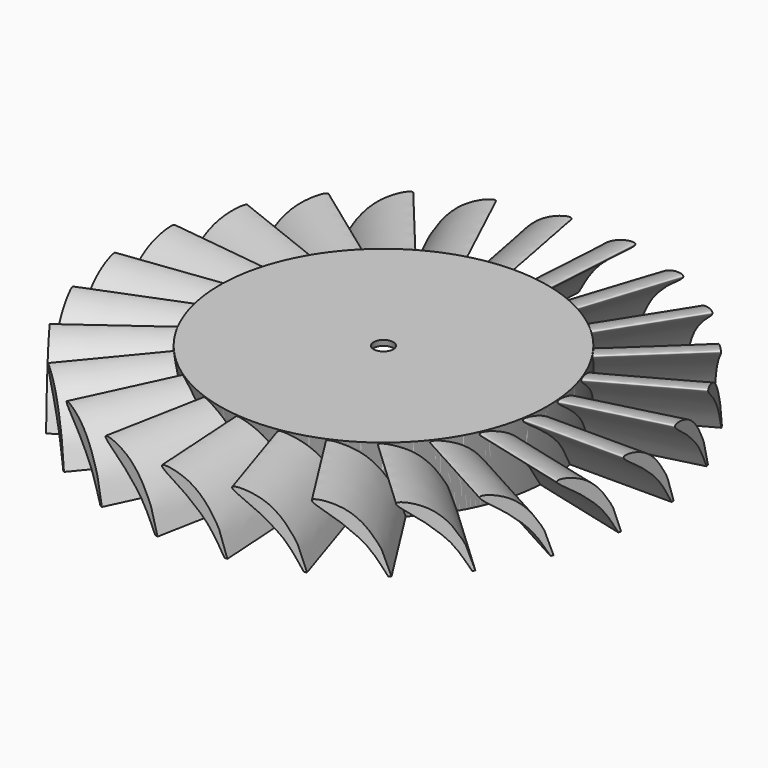
from build123d import *

# Parameters (mm, degrees)
F0_R     = 25
F0_R_2   = 1.5
F1_DEPTH = 10
F4_DEPTH = 15.5780318428
F5_COUNT = 25
F6_R     = 24.6
F6_R_2   = 1.5
F7_DEPTH = 9.2


with BuildPart() as f1:
    # F0 (on Top) → F1 (new body)
    with BuildSketch(Plane.XY):
        Circle(F0_R)
        Circle(F0_R_2, mode=Mode.SUBTRACT)
    extrude(amount=F1_DEPTH)

    # F3 (on offset) → F4 (join, through all)
    with BuildSketch(Plane.YZ.offset(40)):
        with BuildLine():
            add(Edge.make_bspline(
                [(5.3448542021, 0), (4.2896647938, 3.3400247339), (4.3254905267, 3.4207163837), (0.9063081363, 9.1748341728), (-5.955436583, 10.4542680782), (-1.3194624465, 7.5467412737), (2.171653313, 4.4080313078), (3.2502382985, 2.9565140213), (4.9448542021, 0)],
                knots=[0, 0, 0, 0, 0.1648717746, 0.3504462823, 0.5117291158, 0.6489396329, 0.8151774316, 1, 1, 1, 1], degree=3))
            Line((4.9448542021, 0), (5.3448542021, 0))
        make_face()
    extrude(amount=-F4_DEPTH)


with BuildPart() as f5_1:
    # F5: instance of F1
    add(f1.part.rotate(Axis((0, 0, 0), (0, 0, -1)), 1 * 360 / F5_COUNT))


with BuildPart() as f5_2:
    # F5: instance of F1
    add(f1.part.rotate(Axis((0, 0, 0), (0, 0, -1)), 2 * 360 / F5_COUNT))


with BuildPart() as f5_3:
    # F5: instance of F1
    add(f1.part.rotate(Axis((0, 0, 0), (0, 0, -1)), 3 * 360 / F5_COUNT))


with BuildPart() as f5_4:
    # F5: instance of F1
    add(f1.part.rotate(Axis((0, 0, 0), (0, 0, -1)), 4 * 360 / F5_COUNT))


with BuildPart() as f5_5:
    # F5: instance of F1
    add(f1.part.rotate(Axis((0, 0, 0), (0, 0, -1)), 5 * 360 / F5_COUNT))


with BuildPart() as f5_6:
    # F5: instance of F1
    add(f1.part.rotate(Axis((0, 0, 0), (0, 0, -1)), 6 * 360 / F5_COUNT))


with BuildPart() as f5_7:
    # F5: instance of F1
    add(f1.part.rotate(Axis((0, 0, 0), (0, 0, -1)), 7 * 360 / F5_COUNT))


with BuildPart() as f5_8:
    # F5: instance of F1
    add(f1.part.rotate(Axis((0, 0, 0), (0, 0, -1)), 8 * 360 / F5_COUNT))


with BuildPart() as f5_9:
    # F5: instance of F1
    add(f1.part.rotate(Axis((0, 0, 0), (0, 0, -1)), 9 * 360 / F5_COUNT))


with BuildPart() as f5_10:
    # F5: instance of F1
    add(f1.part.rotate(Axis((0, 0, 0), (0, 0, -1)), 10 * 360 / F5_COUNT))


with BuildPart() as f5_11:
    # F5: instance of F1
    add(f1.part.rotate(Axis((0, 0, 0), (0, 0, -1)), 11 * 360 / F5_COUNT))


with BuildPart() as f5_12:
    # F5: instance of F1
    add(f1.part.rotate(Axis((0, 0, 0), (0, 0, -1)), 12 * 360 / F5_COUNT))


with BuildPart() as f5_13:
    # F5: instance of F1
    add(f1.part.rotate(Axis((0, 0, 0), (0, 0, -1)), 13 * 360 / F5_COUNT))


with BuildPart() as f5_14:
    # F5: instance of F1
    add(f1.part.rotate(Axis((0, 0, 0), (0, 0, -1)), 14 * 360 / F5_COUNT))


with BuildPart() as f5_15:
    # F5: instance of F1
    add(f1.part.rotate(Axis((0, 0, 0), (0, 0, -1)), 15 * 360 / F5_COUNT))


with BuildPart() as f5_16:
    # F5: instance of F1
    add(f1.part.rotate(Axis((0, 0, 0), (0, 0, -1)), 16 * 360 / F5_COUNT))


with BuildPart() as f5_17:
    # F5: instance of F1
    add(f1.part.rotate(Axis((0, 0, 0), (0, 0, -1)), 17 * 360 / F5_COUNT))


with BuildPart() as f5_18:
    # F5: instance of F1
    add(f1.part.rotate(Axis((0, 0, 0), (0, 0, -1)), 18 * 360 / F5_COUNT))


with BuildPart() as f5_19:
    # F5: instance of F1
    add(f1.part.rotate(Axis((0, 0, 0), (0, 0, -1)), 19 * 360 / F5_COUNT))


with BuildPart() as f5_20:
    # F5: instance of F1
    add(f1.part.rotate(Axis((0, 0, 0), (0, 0, -1)), 20 * 360 / F5_COUNT))


with BuildPart() as f5_21:
    # F5: instance of F1
    add(f1.part.rotate(Axis((0, 0, 0), (0, 0, -1)), 21 * 360 / F5_COUNT))


with BuildPart() as f5_22:
    # F5: instance of F1
    add(f1.part.rotate(Axis((0, 0, 0), (0, 0, -1)), 22 * 360 / F5_COUNT))


with BuildPart() as f5_23:
    # F5: instance of F1
    add(f1.part.rotate(Axis((0, 0, 0), (0, 0, -1)), 23 * 360 / F5_COUNT))


with BuildPart() as f5_24:
    # F5: instance of F1
    add(f1.part.rotate(Axis((0, 0, 0), (0, 0, -1)), 24 * 360 / F5_COUNT))


with BuildPart() as f7_tool:
    # F6 (on face) → F7 (new body)
    with BuildSketch(Plane(origin=(0, 0, 0), x_dir=(1, 0, 0), z_dir=(0, 0, -1))):
        Circle(F6_R)
        Circle(F6_R_2, mode=Mode.SUBTRACT)
    extrude(amount=-F7_DEPTH)


with BuildPart() as f1_1:
    add(f1.part)

    # F7: cut by f7_tool
    add(f7_tool.part, mode=Mode.SUBTRACT)


with BuildPart() as f5_1_1:
    add(f5_1.part)

    # F7: cut by f7_tool
    add(f7_tool.part, mode=Mode.SUBTRACT)


with BuildPart() as f5_2_1:
    add(f5_2.part)

    # F7: cut by f7_tool
    add(f7_tool.part, mode=Mode.SUBTRACT)


with BuildPart() as f5_3_1:
    add(f5_3.part)

    # F7: cut by f7_tool
    add(f7_tool.part, mode=Mode.SUBTRACT)


with BuildPart() as f5_4_1:
    add(f5_4.part)

    # F7: cut by f7_tool
    add(f7_tool.part, mode=Mode.SUBTRACT)


with BuildPart() as f5_5_1:
    add(f5_5.part)

    # F7: cut by f7_tool
    add(f7_tool.part, mode=Mode.SUBTRACT)


with BuildPart() as f5_6_1:
    add(f5_6.part)

    # F7: cut by f7_tool
    add(f7_tool.part, mode=Mode.SUBTRACT)


with BuildPart() as f5_7_1:
    add(f5_7.part)

    # F7: cut by f7_tool
    add(f7_tool.part, mode=Mode.SUBTRACT)


with BuildPart() as f5_8_1:
    add(f5_8.part)

    # F7: cut by f7_tool
    add(f7_tool.part, mode=Mode.SUBTRACT)


with BuildPart() as f5_9_1:
    add(f5_9.part)

    # F7: cut by f7_tool
    add(f7_tool.part, mode=Mode.SUBTRACT)


with BuildPart() as f5_10_1:
    add(f5_10.part)

    # F7: cut by f7_tool
    add(f7_tool.part, mode=Mode.SUBTRACT)


with BuildPart() as f5_11_1:
    add(f5_11.part)

    # F7: cut by f7_tool
    add(f7_tool.part, mode=Mode.SUBTRACT)


with BuildPart() as f5_12_1:
    add(f5_12.part)

    # F7: cut by f7_tool
    add(f7_tool.part, mode=Mode.SUBTRACT)


with BuildPart() as f5_13_1:
    add(f5_13.part)

    # F7: cut by f7_tool
    add(f7_tool.part, mode=Mode.SUBTRACT)


with BuildPart() as f5_14_1:
    add(f5_14.part)

    # F7: cut by f7_tool
    add(f7_tool.part, mode=Mode.SUBTRACT)


with BuildPart() as f5_15_1:
    add(f5_15.part)

    # F7: cut by f7_tool
    add(f7_tool.part, mode=Mode.SUBTRACT)


with BuildPart() as f5_16_1:
    add(f5_16.part)

    # F7: cut by f7_tool
    add(f7_tool.part, mode=Mode.SUBTRACT)


with BuildPart() as f5_17_1:
    add(f5_17.part)

    # F7: cut by f7_tool
    add(f7_tool.part, mode=Mode.SUBTRACT)


with BuildPart() as f5_18_1:
    add(f5_18.part)

    # F7: cut by f7_tool
    add(f7_tool.part, mode=Mode.SUBTRACT)


with BuildPart() as f5_19_1:
    add(f5_19.part)

    # F7: cut by f7_tool
    add(f7_tool.part, mode=Mode.SUBTRACT)


with BuildPart() as f5_20_1:
    add(f5_20.part)

    # F7: cut by f7_tool
    add(f7_tool.part, mode=Mode.SUBTRACT)


with BuildPart() as f5_21_1:
    add(f5_21.part)

    # F7: cut by f7_tool
    add(f7_tool.part, mode=Mode.SUBTRACT)


with BuildPart() as f5_22_1:
    add(f5_22.part)

    # F7: cut by f7_tool
    add(f7_tool.part, mode=Mode.SUBTRACT)


with BuildPart() as f5_23_1:
    add(f5_23.part)

    # F7: cut by f7_tool
    add(f7_tool.part, mode=Mode.SUBTRACT)


with BuildPart() as f5_24_1:
    add(f5_24.part)

    # F7: cut by f7_tool
    add(f7_tool.part, mode=Mode.SUBTRACT)


solid = Compound([f1_1.part, f5_1_1.part, f5_2_1.part, f5_3_1.part, f5_4_1.part, f5_5_1.part, f5_6_1.part, f5_7_1.part, f5_8_1.part, f5_9_1.part, f5_10_1.part, f5_11_1.part, f5_12_1.part, f5_13_1.part, f5_14_1.part, f5_15_1.part, f5_16_1.part, f5_17_1.part, f5_18_1.part, f5_19_1.part, f5_20_1.part, f5_21_1.part, f5_22_1.part, f5_23_1.part, f5_24_1.part])
